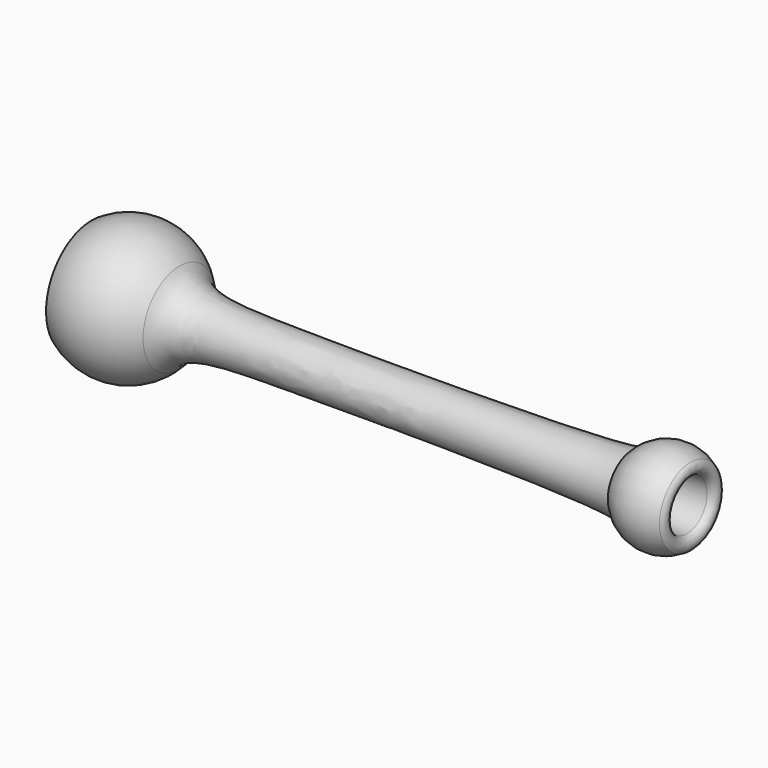
from build123d import *

# Parameters (mm, degrees)
F2_R = 2


# Not quite as in the source:
# - a fillet or chamfer that OpenCascade refuses, or shapes differently, is made with other operations: its cross-section is extruded or revolved along the edge and cut away or added


with BuildPart() as f1:
    # F0 (on Front) → F1 (revolve)
    with BuildSketch(Plane.XZ):
        with BuildLine():
            ThreePointArc((-7.0685046336, 10.3095219212), (4.6853520259, 11.5886788028), (12.2474487139, 2.5))
            Line((12.2474487139, 2.5), (74.2474487139, 2.5))
            Line((74.2474487139, 2.5), (156.0872918181, 7.1431916891))
            ThreePointArc((156.0872918181, 7.1431916891), (146.8168208834, 12.5435983185), (136.9325101955, 8.371497488))
            add(Edge.make_bspline(
                [(13.7809895682, 12.3177978136), (17.0809857804, 6.8756798123), (43.2263367393, 6.4086219424), (128.3770948763, 6.3639083958), (136.9325101955, 8.371497488)],
                knots=[0, 0, 0, 0, 0.3655952784, 1, 1, 1, 1], degree=3))
            ThreePointArc((13.7809895682, 12.3177978136), (2.4835532955, 18.3159979112), (-10.003236638, 15.5428141988))
            Line((-10.003236638, 15.5428141988), (-7.0685046336, 10.3095219212))
        make_face()
    revolve(axis=Axis((35, 0, 0), (1, 0, 0)))

    # F2
    f2_edges = [f1.edges().sort_by_distance(p)[0] for p in [
        (156.087292, 0, -7.143192),
        (-7.068505, 0, -10.309522),
        (12.247449, 0, -2.5),
    ]]
    fillet(f2_edges, radius=F2_R)

    # F3: fillet of radius 5 on 1 edges, made by hand

    # F3_s1 → F3_t2 (revolve, cut)
    with BuildSketch(Plane.XZ):
        with BuildLine():
            ThreePointArc((74.3889449619, 2.5080278038), (74.247391816, 2.5020073539), (74.1057249198, 2.5))
            Line((74.1057249198, 2.5), (74.1057249198, 2.4))
            Line((74.1057249198, 2.4), (74.2502831898, 2.4))
            Line((74.2502831898, 2.4), (74.3946093628, 2.4081883599))
            Line((74.3946093628, 2.4081883599), (74.3889449619, 2.5080278038))
        make_face()
    revolve(axis=Axis((74.2474487139, 0, 0), (1, 0, 0)), mode=Mode.SUBTRACT)


solid = f1.part
